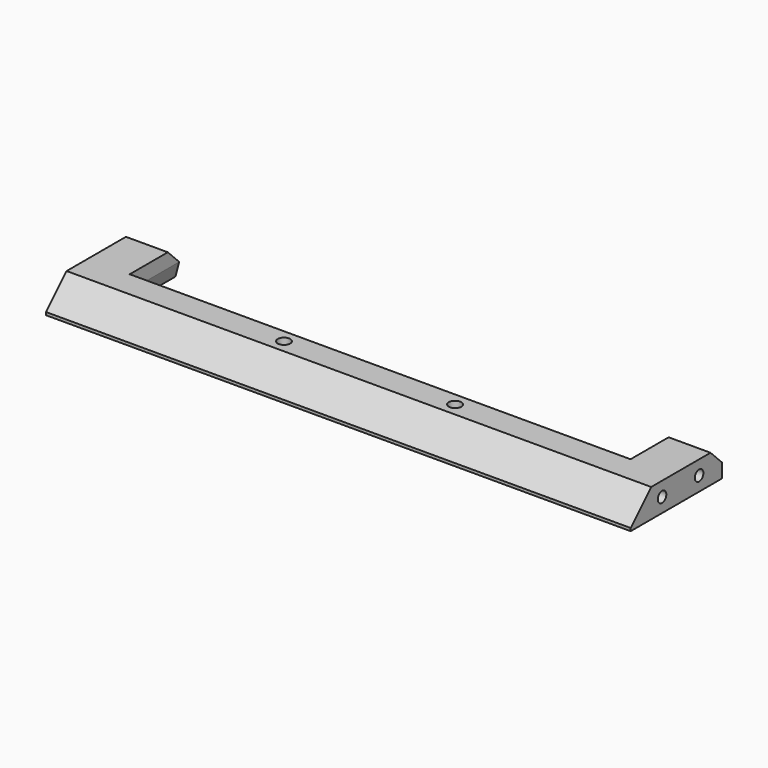
from build123d import *

# Parameters (mm, degrees)
F0_W      = 520.7
F0_H      = 101.6
F1_DEPTH  = 25.4
F2_SIZE   = 22.86
F3_W      = 446.0748
F3_H      = 55.118
F4_DEPTH  = 25.401
F6_DEPTH  = 55.118
F7_SIZE   = 12.7
F9_DEPTH  = 228.6
F10_R     = 5.55625
F11_DEPTH = 6.35
F12_R     = 4.7625
F13_DEPTH = 19.05
F15_DEPTH = 224.028
F16_R     = 0.81661


# Not quite as in the source:
# - a pattern or mirror of a feature is missing from the dataset's text; its kind, count and spacing are read off the source's solid


with BuildPart() as f1:
    # F0 (on Top) → F1 (new body)
    with BuildSketch(Plane.XY):
        with Locations((0, 50.8)):
            Rectangle(F0_W, F0_H)
    extrude(amount=F1_DEPTH)

    # F2
    f2_edges = [f1.edges().sort_by_distance(p)[0] for p in [
        (0, 0, 25.4),
    ]]
    chamfer(f2_edges, length=F2_SIZE)

    # F3 (on face) → F4 (cut, through all)
    with BuildSketch(Plane.XY.offset(25.4)):
        with Locations((0, 74.041)):
            Rectangle(F3_W, F3_H)
    extrude(amount=-F4_DEPTH, mode=Mode.SUBTRACT)

    # F5 (on face) → F6 (cut, through all)
    with BuildSketch(Plane(origin=(0, 101.6, 0), x_dir=(-1, 0, 0), z_dir=(0, 1, 0))):
        Polygon((-223.0374, 0), (-223.0374, 12.7), (-226.4403547439, 0), align=None)
        Polygon((223.0374, 0), (226.4403547439, 0), (223.0374, 12.7), align=None)
    extrude(amount=-F6_DEPTH, mode=Mode.SUBTRACT)

    # F7
    f7_edges = [f1.edges().sort_by_distance(p)[0] for p in [
        (241.6937, 101.6, 25.4),
        (-241.6937, 101.6, 25.4),
    ]]
    chamfer(f7_edges, length=F7_SIZE)

    # F8 (on Right) → F9 (join, symmetric)
    with BuildSketch(Plane.YZ):
        Polygon((71.0692, 0.8128), (46.482, 25.4), (46.482, 0), (71.0692, 0), align=None)
    extrude(amount=F9_DEPTH, both=True)

    # F10 (on face) → F11 (cut)
    with BuildSketch(Plane.XY.offset(25.4)):
        with Locations((76.2, 34.671)):
            Circle(F10_R)
        with Locations((-76.2, 34.671)):
            Circle(F10_R)
    extrude(amount=-F11_DEPTH, mode=Mode.SUBTRACT)

    # F12 (on face) → F13 (cut)
    with BuildSketch(Plane.YZ.offset(260.35)):
        with Locations((34.925, 12.7)):
            Circle(F12_R)
        with Locations((76.2, 12.7)):
            Circle(F12_R)
    f13 = extrude(amount=-F13_DEPTH, mode=Mode.SUBTRACT)

    # F13_copies: F13 across plane
    add(f13.mirror(Plane(origin=(0, 0, 0), x_dir=(0, 0, -1), z_dir=(-1, 0, 0))), mode=Mode.SUBTRACT)

    # F14 (on Right) → F15 (cut, symmetric)
    with BuildSketch(Plane.YZ):
        Polygon((106.9563822457, 9.3574709382), (0, 0), (107.775054872, 0), align=None)
    extrude(amount=F15_DEPTH, both=True, mode=Mode.SUBTRACT)

    # F16
    f16_edges = [f1.edges().sort_by_distance(p)[0] for p in [
        (0, 66.09908, 5.78292),
    ]]
    fillet(f16_edges, radius=F16_R)


solid = f1.part
